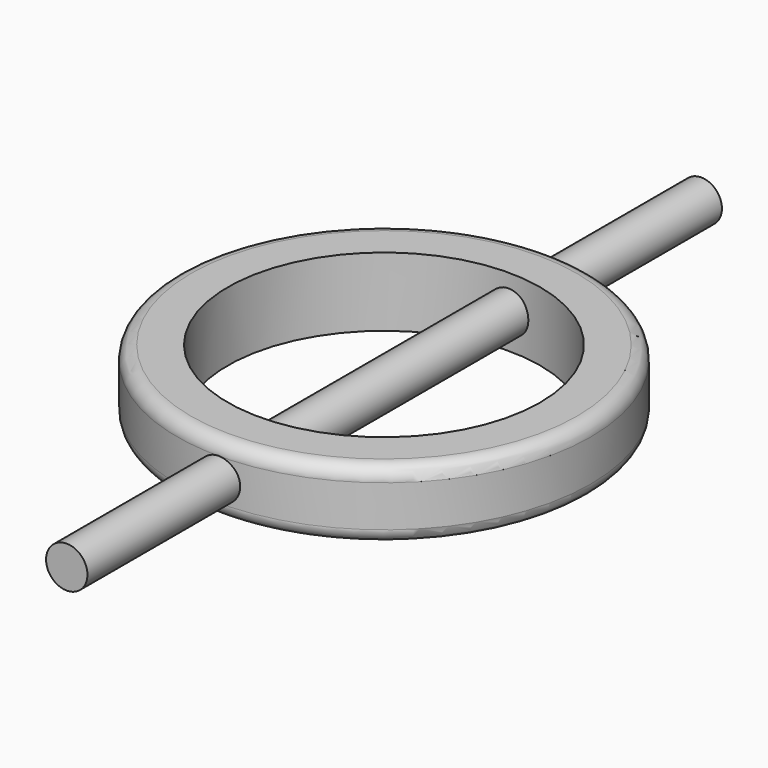
from build123d import *

# Parameters (mm, degrees)
F0_R     = 76.2
F0_R_2   = 57.531
F1_DEPTH = 25.4
F2_R     = 5.08
F3_R     = 7.62
F4_DEPTH = 146.05
F5_DEPTH = 146.05


with BuildPart() as f1:
    # F0 (on Top) → F1 (new body)
    with BuildSketch(Plane.XY):
        Circle(F0_R)
        Circle(F0_R_2, mode=Mode.SUBTRACT)
    extrude(amount=F1_DEPTH)

    # F2
    f2_edges = [f1.edges().sort_by_distance(p)[0] for p in [
        (-76.2, 0, 25.4),
        (-76.2, 0, 0),
    ]]
    fillet(f2_edges, radius=F2_R)


with BuildPart() as f4:
    # F3 (on Front) → F4 (new body)
    with BuildSketch(Plane.XZ):
        with Locations((0, 12.7)):
            Circle(F3_R)
    extrude(amount=F4_DEPTH)

    # F5 (add): a face of the model
    f5_faces = [f4.faces().sort_by_distance(p)[0] for p in [
        (0, 0, 12.7),
    ]]
    extrude(f5_faces, amount=F5_DEPTH)


solid = Compound([f1.part, f4.part])
